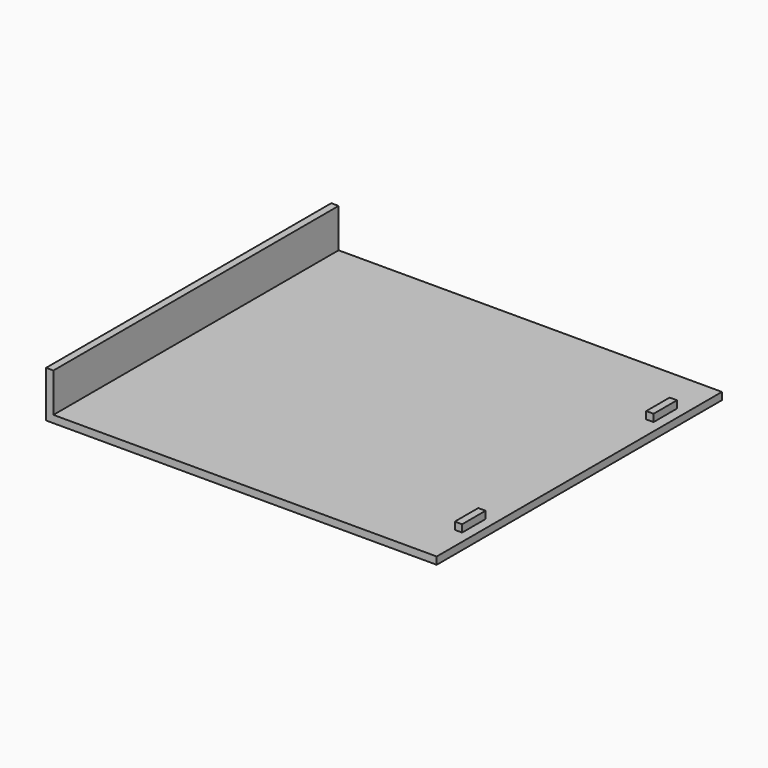
from build123d import *

# Parameters (mm, degrees)
F0_W     = 152.4
F0_H     = 231.775
F0_W_2   = 25.4
F0_W_3   = 76.2
F1_DEPTH = 4.7625
F2_W     = 4.7625
F2_H     = 231.775
F3_DEPTH = 25.4
F4_W     = 4.7625
F4_H     = 9.525
F5_DEPTH = 9.525


with BuildPart() as f1:
    # F0 (on Top) → F1 (new body)
    with BuildSketch(Plane.XY):
        Rectangle(F0_W, F0_H)
        with Locations((-88.9, 0)):
            Rectangle(F0_W_2, F0_H)
        with Locations((-139.7, 0)):
            Rectangle(F0_W_3, F0_H)
    extrude(amount=F1_DEPTH)

    # F2 (on face) → F3 (join)
    with BuildSketch(Plane.XY.offset(4.7625)):
        with Locations((-175.41875, 0)):
            Rectangle(F2_W, F2_H)
    extrude(amount=F3_DEPTH)

    # F4 (on face) → F5 (join)
    with BuildSketch(Plane(origin=(0, 0, 0), x_dir=(1, 0, 0), z_dir=(0, 0, -1))):
        with Locations((67.46875, 73.025)):
            Rectangle(F4_W, F4_H)
        with Locations((67.46875, -73.025)):
            Rectangle(F4_W, F4_H)
        with Locations((67.46875, 82.55)):
            Rectangle(F4_W, F4_H)
        with Locations((67.46875, -82.55)):
            Rectangle(F4_W, F4_H)
    extrude(amount=-F5_DEPTH)


solid = f1.part
